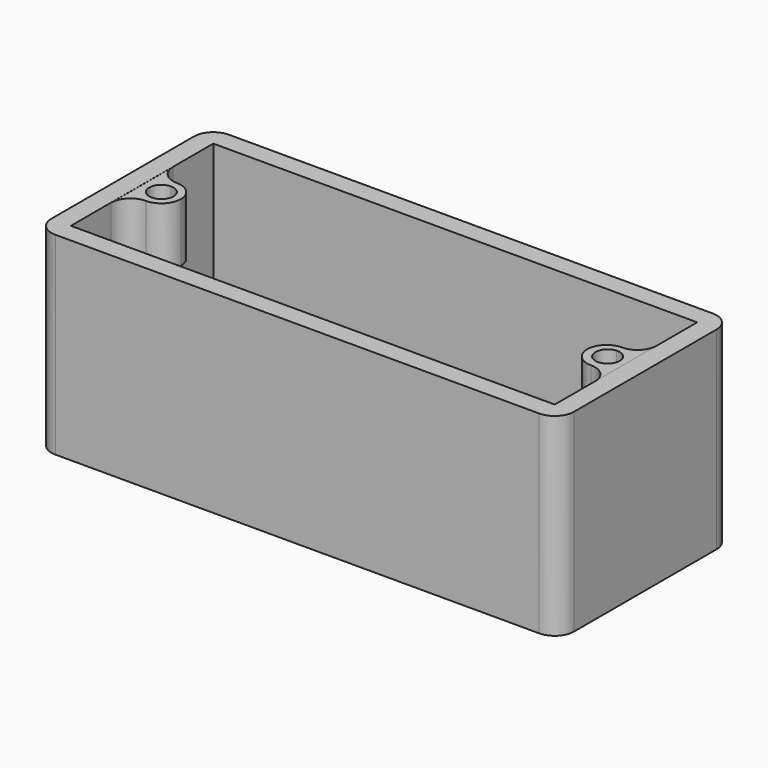
from build123d import *

# Parameters (mm, degrees)
F0_W     = 54
F0_H     = 22.4
F1_DEPTH = 20
F0_W_2   = 5
F0_H_2   = 5
F0_W_3   = 1.5
F0_H_3   = 1.5
F2_DEPTH = 2
F4_START = -20.2
F3_W     = 9
F3_H     = 6
F4_DEPTH = 15.6
F5_DEPTH = 10
F6_START = 13.91
F6_DEPTH = 6.08
F7_R     = 1.99999
F8_DEPTH = 6


# Not quite as in the source:
# - a fillet or chamfer is up to 0.001 mm smaller than in the source, because OpenCascade refuses the exact size


with BuildPart() as f1:
    # F0 (on Top) → F1 (new body)
    with BuildSketch(Plane.XY):
        with Locations((-4.5801811367, 0)):
            Rectangle(F0_W, F0_H)
        Polygon((-29.5801811367, 7.7), (-29.5801811367, 9.2), (-28.0801811367, 9.2), (13.2198188633, 9.2), (14.7198188633, 9.2), (20.4198188633, 9.2), (20.4198188633, 2), (20.4198188633, 0), (20.4198188633, -2), (20.4198188633, -9.2), (14.7198188633, -9.2), (13.2198188633, -9.2), (-28.0801811367, -9.2), (-29.5801811367, -9.2), (-29.5801811367, -7.7), (-29.5801811367, -2), (-29.5801811367, 0), (-29.5801811367, 2), align=None, mode=Mode.SUBTRACT)
    extrude(amount=F1_DEPTH)

    # F0 (on Top) → F2 (join)
    with BuildSketch(Plane.XY):
        with BuildLine():
            Line((20.4198188633, 9.2), (14.7198188633, 9.2))
            Line((14.7198188633, 9.2), (14.7198188633, 7.7))
            Line((14.7198188633, 7.7), (14.7198188633, -7.7))
            Line((14.7198188633, -7.7), (14.7198188633, -9.2))
            Line((14.7198188633, -9.2), (20.4198188633, -9.2))
            Line((20.4198188633, -9.2), (20.4198188633, -2))
            Line((20.4198188633, -2), (18.4198188633, -2))
            ThreePointArc((18.4198188633, -2), (16.4198188633, 0), (18.4198188633, 2))
            Line((18.4198188633, 2), (20.4198188633, 2))
            Line((20.4198188633, 2), (20.4198188633, 9.2))
        make_face()
        with BuildLine():
            Line((13.2198188633, 9.2), (-28.0801811367, 9.2))
            Line((-28.0801811367, 9.2), (-28.0801811367, 7.7))
            Line((-28.0801811367, 7.7), (-29.5801811367, 7.7))
            Line((-29.5801811367, 7.7), (-29.5801811367, 2))
            Line((-29.5801811367, 2), (-27.5801811367, 2))
            ThreePointArc((-27.5801811367, 2), (-26.1659675744, 1.4142135624), (-25.5801811367, 0))
            ThreePointArc((-25.5801811367, 0), (-26.1659675744, -1.4142135624), (-27.5801811367, -2))
            Line((-27.5801811367, -2), (-29.5801811367, -2))
            Line((-29.5801811367, -2), (-29.5801811367, -7.7))
            Line((-29.5801811367, -7.7), (-28.0801811367, -7.7))
            Line((-28.0801811367, -7.7), (-28.0801811367, -9.2))
            Line((-28.0801811367, -9.2), (13.2198188633, -9.2))
            Line((13.2198188633, -9.2), (13.2198188633, -7.7))
            Line((13.2198188633, -7.7), (14.7198188633, -7.7))
            Line((14.7198188633, -7.7), (14.7198188633, 7.7))
            Line((14.7198188633, 7.7), (13.2198188633, 7.7))
            Line((13.2198188633, 7.7), (13.2198188633, 9.2))
        make_face()
        with Locations((-5.0801811367, -1.1269363482)):
            Rectangle(F0_W_2, F0_H_2, mode=Mode.SUBTRACT)
        with BuildLine():
            ThreePointArc((18.4198188633, -2), (19.8340324256, -1.4142135624), (20.4198188633, 0))
            ThreePointArc((20.4198188633, 0), (19.8340324256, 1.4142135624), (18.4198188633, 2))
            Line((18.4198188633, 2), (18.4198188633, 1.2932023613))
            ThreePointArc((18.4198188633, 1.2932023613), (19.3476040738, 0.9528353135), (19.7382581234, 0.0450773405))
            ThreePointArc((19.7382581234, 0.0450773405), (19.3476040738, -0.8626806325), (18.4198188633, -1.2030476804))
            Line((18.4198188633, -1.2030476804), (18.4198188633, -2))
        make_face()
        with BuildLine():
            Line((20.4198188633, 0), (20.4198188633, 2))
            Line((20.4198188633, 2), (18.4198188633, 2))
            ThreePointArc((18.4198188633, 2), (19.8340324256, 1.4142135624), (20.4198188633, 0))
        make_face()
        with BuildLine():
            Line((20.4198188633, -2), (20.4198188633, 0))
            ThreePointArc((20.4198188633, 0), (19.8340324256, -1.4142135624), (18.4198188633, -2))
            Line((18.4198188633, -2), (20.4198188633, -2))
        make_face()
        with BuildLine():
            Line((18.4198188633, 1.2932023613), (18.4198188633, 2))
            ThreePointArc((18.4198188633, 2), (16.4198188633, 0), (18.4198188633, -2))
            Line((18.4198188633, -2), (18.4198188633, -1.2030476804))
            ThreePointArc((18.4198188633, -1.2030476804), (17.2382581234, 0.0450773405), (18.4198188633, 1.2932023613))
        make_face()
        with BuildLine():
            Line((18.4198188633, -1.2030476804), (18.4198188633, 1.2932023613))
            ThreePointArc((18.4198188633, 1.2932023613), (17.2382581234, 0.0450773405), (18.4198188633, -1.2030476804))
        make_face()
        with BuildLine():
            ThreePointArc((19.7382581234, 0.0450773405), (19.3476040738, 0.9528353135), (18.4198188633, 1.2932023613))
            Line((18.4198188633, 1.2932023613), (18.4198188633, -1.2030476804))
            ThreePointArc((18.4198188633, -1.2030476804), (19.3476040738, -0.8626806325), (19.7382581234, 0.0450773405))
        make_face()
        with BuildLine():
            Line((-27.5801811367, 2), (-29.5801811367, 2))
            Line((-29.5801811367, 2), (-29.5801811367, 0))
            ThreePointArc((-29.5801811367, 0), (-28.9943946991, 1.4142135624), (-27.5801811367, 2))
        make_face()
        with BuildLine():
            ThreePointArc((-27.5801811367, -2), (-28.9943946991, -1.4142135624), (-29.5801811367, 0))
            Line((-29.5801811367, 0), (-29.5801811367, -2))
            Line((-29.5801811367, -2), (-27.5801811367, -2))
        make_face()
        with BuildLine():
            ThreePointArc((-27.5801811367, 2), (-28.9943946991, 1.4142135624), (-29.5801811367, 0))
            ThreePointArc((-29.5801811367, 0), (-28.9943946991, -1.4142135624), (-27.5801811367, -2))
            Line((-27.5801811367, -2), (-27.5801811367, -1.25))
            ThreePointArc((-27.5801811367, -1.25), (-28.8301811367, 0), (-27.5801811367, 1.25))
            Line((-27.5801811367, 1.25), (-27.5801811367, 2))
        make_face()
        with BuildLine():
            ThreePointArc((-25.5801811367, 0), (-26.1659675744, 1.4142135624), (-27.5801811367, 2))
            Line((-27.5801811367, 2), (-27.5801811367, 1.25))
            ThreePointArc((-27.5801811367, 1.25), (-26.6962976602, 0.8838834765), (-26.3301811367, 0))
            ThreePointArc((-26.3301811367, 0), (-26.6962976602, -0.8838834765), (-27.5801811367, -1.25))
            Line((-27.5801811367, -1.25), (-27.5801811367, -2))
            ThreePointArc((-27.5801811367, -2), (-26.1659675744, -1.4142135624), (-25.5801811367, 0))
        make_face()
        with BuildLine():
            ThreePointArc((-26.3301811367, 0), (-26.6962976602, 0.8838834765), (-27.5801811367, 1.25))
            Line((-27.5801811367, 1.25), (-27.5801811367, -1.25))
            ThreePointArc((-27.5801811367, -1.25), (-26.6962976602, -0.8838834765), (-26.3301811367, 0))
        make_face()
        with BuildLine():
            Line((-27.5801811367, -1.25), (-27.5801811367, 1.25))
            ThreePointArc((-27.5801811367, 1.25), (-28.8301811367, 0), (-27.5801811367, -1.25))
        make_face()
        with Locations((-5.0801811367, -1.1269363482)):
            Rectangle(F0_W_2, F0_H_2)
        with Locations((-28.8301811367, 8.45)):
            Rectangle(F0_W_3, F0_H_3)
        with Locations((-28.8301811367, -8.45)):
            Rectangle(F0_W_3, F0_H_3)
        with Locations((13.9698188633, 8.45)):
            Rectangle(F0_W_3, F0_H_3)
        with Locations((13.9698188633, -8.45)):
            Rectangle(F0_W_3, F0_H_3)
    extrude(amount=F2_DEPTH)

    # F3 (on Right) → F4 (cut)
    with BuildSketch(Plane.YZ.offset(F4_START)):
        with Locations((0.2, 9)):
            Rectangle(F3_W, F3_H)
    extrude(amount=-F4_DEPTH, mode=Mode.SUBTRACT)

    # F0 (on Top) → F5 (join)
    with BuildSketch(Plane.XY):
        with BuildLine():
            Line((18.4198188633, 1.2932023613), (18.4198188633, 2))
            ThreePointArc((18.4198188633, 2), (16.4198188633, 0), (18.4198188633, -2))
            Line((18.4198188633, -2), (18.4198188633, -1.2030476804))
            ThreePointArc((18.4198188633, -1.2030476804), (17.2382581234, 0.0450773405), (18.4198188633, 1.2932023613))
        make_face()
        with BuildLine():
            Line((18.4198188633, -1.2030476804), (18.4198188633, 1.2932023613))
            ThreePointArc((18.4198188633, 1.2932023613), (17.2382581234, 0.0450773405), (18.4198188633, -1.2030476804))
        make_face()
        with BuildLine():
            ThreePointArc((19.7382581234, 0.0450773405), (19.3476040738, 0.9528353135), (18.4198188633, 1.2932023613))
            Line((18.4198188633, 1.2932023613), (18.4198188633, -1.2030476804))
            ThreePointArc((18.4198188633, -1.2030476804), (19.3476040738, -0.8626806325), (19.7382581234, 0.0450773405))
        make_face()
        with BuildLine():
            ThreePointArc((18.4198188633, -2), (19.8340324256, -1.4142135624), (20.4198188633, 0))
            ThreePointArc((20.4198188633, 0), (19.8340324256, 1.4142135624), (18.4198188633, 2))
            Line((18.4198188633, 2), (18.4198188633, 1.2932023613))
            ThreePointArc((18.4198188633, 1.2932023613), (19.3476040738, 0.9528353135), (19.7382581234, 0.0450773405))
            ThreePointArc((19.7382581234, 0.0450773405), (19.3476040738, -0.8626806325), (18.4198188633, -1.2030476804))
            Line((18.4198188633, -1.2030476804), (18.4198188633, -2))
        make_face()
        with BuildLine():
            Line((20.4198188633, 0), (20.4198188633, 2))
            Line((20.4198188633, 2), (18.4198188633, 2))
            ThreePointArc((18.4198188633, 2), (19.8340324256, 1.4142135624), (20.4198188633, 0))
        make_face()
        with BuildLine():
            Line((20.4198188633, -2), (20.4198188633, 0))
            ThreePointArc((20.4198188633, 0), (19.8340324256, -1.4142135624), (18.4198188633, -2))
            Line((18.4198188633, -2), (20.4198188633, -2))
        make_face()
        with BuildLine():
            Line((20.4198188633, 9.2), (14.7198188633, 9.2))
            Line((14.7198188633, 9.2), (14.7198188633, 7.7))
            Line((14.7198188633, 7.7), (14.7198188633, -7.7))
            Line((14.7198188633, -7.7), (14.7198188633, -9.2))
            Line((14.7198188633, -9.2), (20.4198188633, -9.2))
            Line((20.4198188633, -9.2), (20.4198188633, -2))
            Line((20.4198188633, -2), (18.4198188633, -2))
            ThreePointArc((18.4198188633, -2), (16.4198188633, 0), (18.4198188633, 2))
            Line((18.4198188633, 2), (20.4198188633, 2))
            Line((20.4198188633, 2), (20.4198188633, 9.2))
        make_face()
    extrude(amount=F5_DEPTH)

    # F0 (on Top) → F6 (join)
    with BuildSketch(Plane.XY.offset(F6_START)):
        with BuildLine():
            Line((20.4198188633, 0), (20.4198188633, 2))
            Line((20.4198188633, 2), (18.4198188633, 2))
            ThreePointArc((18.4198188633, 2), (19.8340324256, 1.4142135624), (20.4198188633, 0))
        make_face()
        with BuildLine():
            ThreePointArc((18.4198188633, -2), (19.8340324256, -1.4142135624), (20.4198188633, 0))
            ThreePointArc((20.4198188633, 0), (19.8340324256, 1.4142135624), (18.4198188633, 2))
            Line((18.4198188633, 2), (18.4198188633, 1.2932023613))
            ThreePointArc((18.4198188633, 1.2932023613), (19.3476040738, 0.9528353135), (19.7382581234, 0.0450773405))
            ThreePointArc((19.7382581234, 0.0450773405), (19.3476040738, -0.8626806325), (18.4198188633, -1.2030476804))
            Line((18.4198188633, -1.2030476804), (18.4198188633, -2))
        make_face()
        with BuildLine():
            Line((20.4198188633, -2), (20.4198188633, 0))
            ThreePointArc((20.4198188633, 0), (19.8340324256, -1.4142135624), (18.4198188633, -2))
            Line((18.4198188633, -2), (20.4198188633, -2))
        make_face()
        with BuildLine():
            Line((18.4198188633, 1.2932023613), (18.4198188633, 2))
            ThreePointArc((18.4198188633, 2), (16.4198188633, 0), (18.4198188633, -2))
            Line((18.4198188633, -2), (18.4198188633, -1.2030476804))
            ThreePointArc((18.4198188633, -1.2030476804), (17.2382581234, 0.0450773405), (18.4198188633, 1.2932023613))
        make_face()
        with BuildLine():
            Line((-27.5801811367, 2), (-29.5801811367, 2))
            Line((-29.5801811367, 2), (-29.5801811367, 0))
            ThreePointArc((-29.5801811367, 0), (-28.9943946991, 1.4142135624), (-27.5801811367, 2))
        make_face()
        with BuildLine():
            ThreePointArc((-27.5801811367, 2), (-28.9943946991, 1.4142135624), (-29.5801811367, 0))
            ThreePointArc((-29.5801811367, 0), (-28.9943946991, -1.4142135624), (-27.5801811367, -2))
            Line((-27.5801811367, -2), (-27.5801811367, -1.25))
            ThreePointArc((-27.5801811367, -1.25), (-28.8301811367, 0), (-27.5801811367, 1.25))
            Line((-27.5801811367, 1.25), (-27.5801811367, 2))
        make_face()
        with BuildLine():
            ThreePointArc((-25.5801811367, 0), (-26.1659675744, 1.4142135624), (-27.5801811367, 2))
            Line((-27.5801811367, 2), (-27.5801811367, 1.25))
            ThreePointArc((-27.5801811367, 1.25), (-26.6962976602, 0.8838834765), (-26.3301811367, 0))
            ThreePointArc((-26.3301811367, 0), (-26.6962976602, -0.8838834765), (-27.5801811367, -1.25))
            Line((-27.5801811367, -1.25), (-27.5801811367, -2))
            ThreePointArc((-27.5801811367, -2), (-26.1659675744, -1.4142135624), (-25.5801811367, 0))
        make_face()
        with BuildLine():
            ThreePointArc((-27.5801811367, -2), (-28.9943946991, -1.4142135624), (-29.5801811367, 0))
            Line((-29.5801811367, 0), (-29.5801811367, -2))
            Line((-29.5801811367, -2), (-27.5801811367, -2))
        make_face()
    extrude(amount=F6_DEPTH)

    # F7 (radius 2 in the source; OpenCascade refuses exactly that, so slightly less here)
    f7_edges = [f1.edges().sort_by_distance(p)[0] for p in [
        (-31.580181, -11.2, 10),
        (-31.580181, 11.2, 10),
        (22.419819, 11.2, 10),
        (-29.580181, 2, 16.95),
        (-29.580181, -2, 16.95),
        (20.419819, -2, 16.95),
        (20.419819, 2, 16.95),
        (22.419819, -11.2, 10),
    ]]
    fillet(f7_edges, radius=F7_R)

    # F0 (on Top) → F8 (join)
    with BuildSketch(Plane.XY):
        with Locations((-5.0801811367, -1.1269363482)):
            Rectangle(F0_W_2, F0_H_2)
        with Locations((-28.8301811367, 8.45)):
            Rectangle(F0_W_3, F0_H_3)
        with Locations((-28.8301811367, -8.45)):
            Rectangle(F0_W_3, F0_H_3)
        with Locations((13.9698188633, 8.45)):
            Rectangle(F0_W_3, F0_H_3)
        with Locations((13.9698188633, -8.45)):
            Rectangle(F0_W_3, F0_H_3)
    extrude(amount=F8_DEPTH)


solid = f1.part
